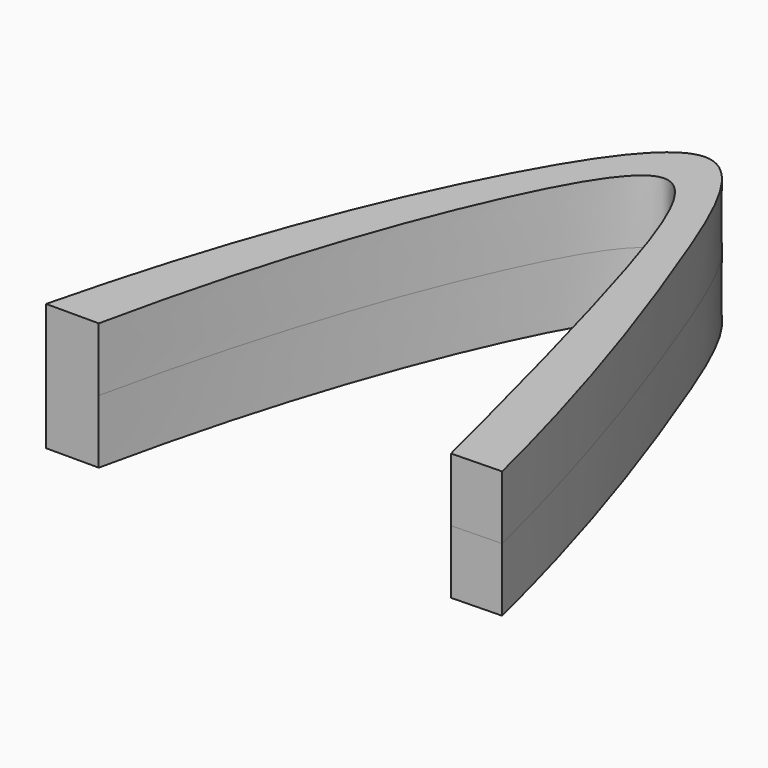
from build123d import *

# Parameters (mm, degrees)
F1_DEPTH = 15.24


with BuildPart() as f1:
    # F0 (on Top) → F1 (new body, symmetric)
    with BuildSketch(Plane.XY):
        with BuildLine():
            add(Edge.make_bspline(
                [(-81.0627639294, -53.9917089045), (-72.5197874696, -19.1585278886), (-54.0247601816, 32.9807166244), (-19.7662531538, 84.9899163352), (3.6253786631, 28.1773385335), (19.5617973002, -19.0915599193), (28.0987489969, -53.6909215152)],
                knots=[0, 0, 0, 0, 0.3075747213, 0.5045905715, 0.700487572, 1, 1, 1, 1], degree=3))
            add(Edge.make_bspline(
                [(-81.0627639294, -53.9917089045), (-76.8517106771, -53.9917089045), (-72.6406574249, -53.9917089045), (-68.4296041727, -53.9917089045)],
                knots=[0, 0, 0, 0, 12.6331597567, 12.6331597567, 12.6331597567, 12.6331597567], degree=3))
            add(Edge.make_bspline(
                [(-68.4296041727, -53.9917089045), (-61.2381206293, -20.2495097403), (-45.6430965514, 28.1570874772), (-21.8702426997, 68.5417920783), (-4.9761473076, 31.8300107745), (15.7164527353, -52.5613601463), (16.0671714693, -53.9917089045)],
                knots=[0, 0, 0, 0, 0.3128036408, 0.4926022052, 0.6780878804, 0.9829136146, 0.9829136146, 0.9829136146, 0.9829136146], degree=3))
            add(Edge.make_bspline(
                [(16.0671714693, -53.9917089045), (19.5847364763, -53.8914464414), (24.5811839898, -53.7911839783), (28.0987489969, -53.6909215152)],
                knots=[0, 0, 0, 0, 12.035336757, 12.035336757, 12.035336757, 12.035336757], degree=3))
        make_face()
    extrude(amount=F1_DEPTH, both=True)


solid = f1.part
